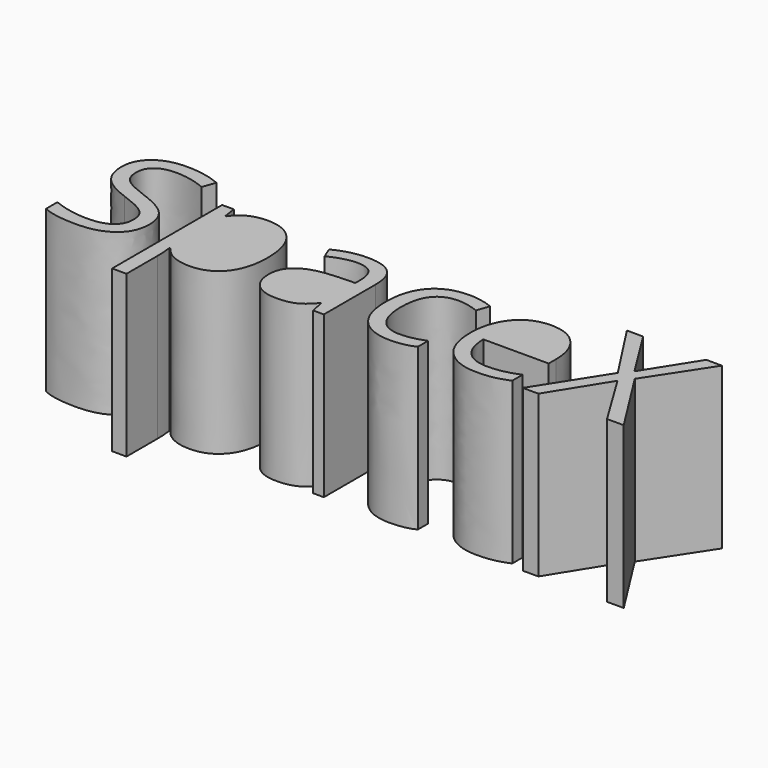
from build123d import *

# Parameters (mm, degrees)
F0_TEXT_SIZE = 27.9802984248
F1_DEPTH     = 25.4


# Not quite as in the source:
# - Text() gives the source's letters only with a copy of the font that has no kerning and outlines rounded to 1/6400 em; it was checked with that copy


with BuildPart() as f1:
    # F0 (on Top) → F1 (new body)
    with BuildSketch(Plane.XY):
        with BuildLine():
            add(Edge.make_bspline(
                [(-34.0867500308, 44.6653611555), (-35.1862883205, 46.1605583526), (-37.1798845833, 46.1605583526)],
                knots=[0, 0, 0, 1, 1, 1], degree=2))
            add(Edge.make_bspline(
                [(-37.1798845833, 46.1605583526), (-39.4751434384, 46.1605583526), (-40.5003590604, 44.8905151194)],
                knots=[0, 0, 0, 1, 1, 1], degree=2))
            add(Edge.make_bspline(
                [(-40.5003590604, 44.8905151194), (-41.5255746824, 43.6204718862), (-41.5518062121, 40.8443016519)],
                knots=[0, 0, 0, 1, 1, 1], degree=2))
            Line((-41.5518062121, 40.8443016519), (-41.5518062121, 40.3415306646))
            add(Edge.make_bspline(
                [(-41.5518062121, 40.3415306646), (-41.5518062121, 37.1850032485), (-40.5003590604, 35.825335622)],
                knots=[0, 0, 0, 1, 1, 1], degree=2))
            add(Edge.make_bspline(
                [(-40.5003590604, 35.825335622), (-39.4489119086, 34.4656679954), (-37.1274215237, 34.4656679954)],
                knots=[0, 0, 0, 1, 1, 1], degree=2))
            add(Edge.make_bspline(
                [(-37.1274215237, 34.4656679954), (-35.1862883205, 34.4656679954), (-34.0867500308, 36.037373821)],
                knots=[0, 0, 0, 1, 1, 1], degree=2))
            add(Edge.make_bspline(
                [(-34.0867500308, 36.037373821), (-32.9872117412, 37.6090796465), (-32.9872117412, 40.3677621944)],
                knots=[0, 0, 0, 1, 1, 1], degree=2))
            add(Edge.make_bspline(
                [(-32.9872117412, 40.3677621944), (-32.9872117412, 43.1701639585), (-34.0867500308, 44.6653611555)],
                knots=[0, 0, 0, 1, 1, 1], degree=2))
        make_face()
        with BuildLine():
            add(Edge.make_bspline(
                [(-24.6718168031, 35.0799229842), (-23.9285901262, 34.4394364656), (-22.5907821077, 34.4394364656)],
                knots=[0, 0, 0, 1, 1, 1], degree=2))
            add(Edge.make_bspline(
                [(-22.5907821077, 34.4394364656), (-20.4704001177, 34.4394364656), (-19.2615637873, 35.6001816581)],
                knots=[0, 0, 0, 1, 1, 1], degree=2))
            add(Edge.make_bspline(
                [(-19.2615637873, 35.6001816581), (-18.052727457, 36.7609268505), (-18.052727457, 38.8507053891)],
                knots=[0, 0, 0, 1, 1, 1], degree=2))
            Line((-18.052727457, 38.8507053891), (-18.052727457, 40.2016291725))
            Line((-18.052727457, 40.2016291725), (-20.3217547823, 40.1098188183))
            add(Edge.make_bspline(
                [(-20.3217547823, 40.1098188183), (-23.0279742706, 40.0136365424), (-24.2215088753, 39.2682239047)],
                knots=[0, 0, 0, 1, 1, 1], degree=2))
            add(Edge.make_bspline(
                [(-24.2215088753, 39.2682239047), (-25.41504348, 38.522811267), (-25.41504348, 36.9532914022)],
                knots=[0, 0, 0, 1, 1, 1], degree=2))
            add(Edge.make_bspline(
                [(-25.41504348, 36.9532914022), (-25.41504348, 35.7204095029), (-24.6718168031, 35.0799229842)],
                knots=[0, 0, 0, 1, 1, 1], degree=2))
        make_face()
        with Locations((-61.5839511156, 32.8393131495)):
            Text('SpaceX', F0_TEXT_SIZE, font='Open Sans', text_align=(TextAlign.LEFT, TextAlign.BOTTOM))
        with BuildLine():
            add(Edge.make_bspline(
                [(10.6511239974, 45.0457183373), (9.6958591215, 46.1867898824), (7.9164870185, 46.1867898824)],
                knots=[0, 0, 0, 1, 1, 1], degree=2))
            add(Edge.make_bspline(
                [(7.9164870185, 46.1867898824), (6.1152553074, 46.1867898824), (5.0419485475, 45.012928925)],
                knots=[0, 0, 0, 1, 1, 1], degree=2))
            add(Edge.make_bspline(
                [(5.0419485475, 45.012928925), (3.9686417877, 43.8390679677), (3.776277236, 41.762405194)],
                knots=[0, 0, 0, 1, 1, 1], degree=2))
            Line((3.776277236, 41.762405194), (11.6063888733, 41.762405194))
            add(Edge.make_bspline(
                [(11.6063888733, 41.762405194), (11.6063888733, 43.9046467921), (10.6511239974, 45.0457183373)],
                knots=[0, 0, 0, 1, 1, 1], degree=2))
        make_face()
    extrude(amount=F1_DEPTH)


solid = f1.part
